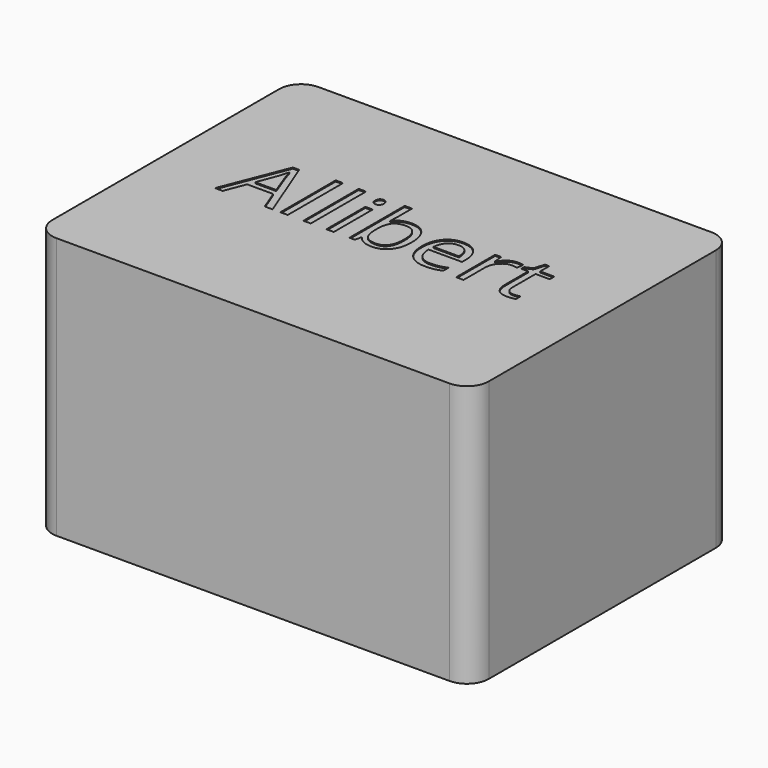
from build123d import *

# Parameters (mm, degrees)
F0_W         = 400
F0_H         = 300
F1_DEPTH     = 240
F2_TEXT_SIZE = 83.3333333333
F3_DEPTH     = 1
F4_R         = 20


# Not quite as in the source:
# - Text() gives the source's letters only with a copy of the font that has no kerning and outlines rounded to 1/6400 em; it was checked with that copy


with BuildPart() as f1:
    # F0 (on Top) → F1 (new body)
    with BuildSketch(Plane.XY):
        Rectangle(F0_W, F0_H)
    extrude(amount=F1_DEPTH)

    # F2 (on face) → F3 (cut)
    with BuildSketch(Plane.XY.offset(240)):
        with Locations((-140, -18.5355305514)):
            Text('Allibert', F2_TEXT_SIZE, font='Open Sans', text_align=(TextAlign.LEFT, TextAlign.BOTTOM))
    extrude(amount=-F3_DEPTH, mode=Mode.SUBTRACT)

    # F4
    f4_edges = [f1.edges().sort_by_distance(p)[0] for p in [
        (-200, -150, 120),
        (-200, 150, 120),
        (200, -150, 120),
        (200, 150, 120),
    ]]
    fillet(f4_edges, radius=F4_R)


solid = f1.part
